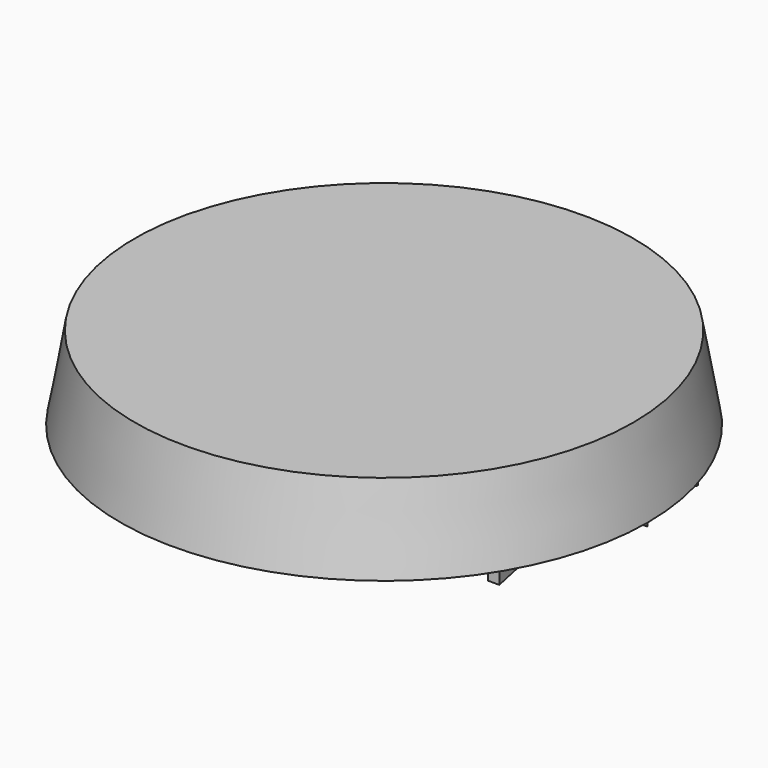
from build123d import *

# Parameters (mm, degrees)
F0_R           = 30
F1_DEPTH       = 10
F1_TAPER       = -10
F2_TEXT_SIZE   = 16.8922161436
F2_TEXT_SIZE_2 = 10.3927492447
F2_TEXT_SIZE_3 = 17.7311169437
F3_DEPTH       = 2


# Not quite as in the source:
# - Text() gives the source's letters only with a copy of the font that has no kerning and outlines rounded to 1/6400 em; it was checked with that copy


with BuildPart() as f1:
    # F0 (on Top) → F1 (new body)
    with BuildSketch(Plane.XY):
        Circle(F0_R)
    extrude(amount=-F1_DEPTH, taper=F1_TAPER)

    # F2 (on face) → F3 (join)
    with BuildSketch(Plane(origin=(0, 0, -10), x_dir=(1, 0, 0), z_dir=(0, 0, -1))):
        with Locations((-27.5, 2.8376043766)):
            Text('God Jul', F2_TEXT_SIZE, font='Open Sans', font_style=FontStyle.ITALIC, text_align=(TextAlign.LEFT, TextAlign.BOTTOM))
        with Locations((-26.5, -10.7664041995)):
            Text('fam.', F2_TEXT_SIZE_2, font='Open Sans', font_style=FontStyle.ITALIC, text_align=(TextAlign.LEFT, TextAlign.BOTTOM))
        with Locations((-7, -11.7664041995)):
            Text('Rask', F2_TEXT_SIZE_3, font='Open Sans', font_style=FontStyle.ITALIC, text_align=(TextAlign.LEFT, TextAlign.BOTTOM))
    extrude(amount=F3_DEPTH)


solid = f1.part
